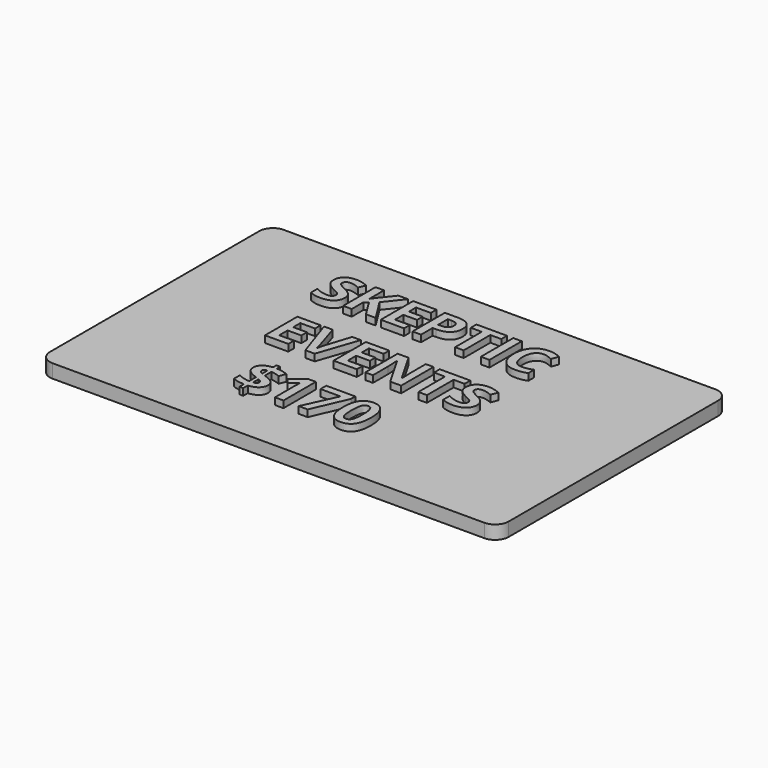
from build123d import *

# Parameters (mm, degrees)
F1_DEPTH     = 2.54
F2_TEXT_SIZE = 10.5833333333
F3_DEPTH     = 1.27


# Not quite as in the source:
# - Text() gives the source's letters only with a copy of the font that has no kerning and outlines rounded to 1/6400 em; it was checked with that copy


with BuildPart() as f1:
    # F0 (on Top) → F1 (new body)
    with BuildSketch(Plane.XY):
        with BuildLine():
            ThreePointArc((42.8625, 24.4475), (42.1185512242, 26.2435512242), (40.3225, 26.9875))
            Line((40.3225, 26.9875), (-40.3225, 26.9875))
            ThreePointArc((-40.3225, 26.9875), (-42.1185512242, 26.2435512242), (-42.8625, 24.4475))
            Line((-42.8625, 24.4475), (-42.8625, -24.4475))
            ThreePointArc((-42.8625, -24.4475), (-42.1185512242, -26.2435512242), (-40.3225, -26.9875))
            Line((-40.3225, -26.9875), (40.3225, -26.9875))
            ThreePointArc((40.3225, -26.9875), (42.1185512242, -26.2435512242), (42.8625, -24.4475))
            Line((42.8625, -24.4475), (42.8625, 24.4475))
        make_face()
    extrude(amount=F1_DEPTH)

    # F2 (on face) → F3 (join)
    with BuildSketch(Plane.XY.offset(2.54)):
        with Locations((-23.8125, 11.7475)):
            Text('SKEPTIC', F2_TEXT_SIZE, font='Open Sans', font_style=FontStyle.BOLD, text_align=(TextAlign.LEFT, TextAlign.BOTTOM))
        with Locations((-21.0624869792, -2.6458333333)):
            Text('EVENTS', F2_TEXT_SIZE, font='Open Sans', font_style=FontStyle.BOLD, text_align=(TextAlign.LEFT, TextAlign.BOTTOM))
        with Locations((-15.5624609375, -17.0391666667)):
            Text('$170', F2_TEXT_SIZE, font='Open Sans', font_style=FontStyle.BOLD, text_align=(TextAlign.LEFT, TextAlign.BOTTOM))
    extrude(amount=F3_DEPTH)


solid = f1.part
